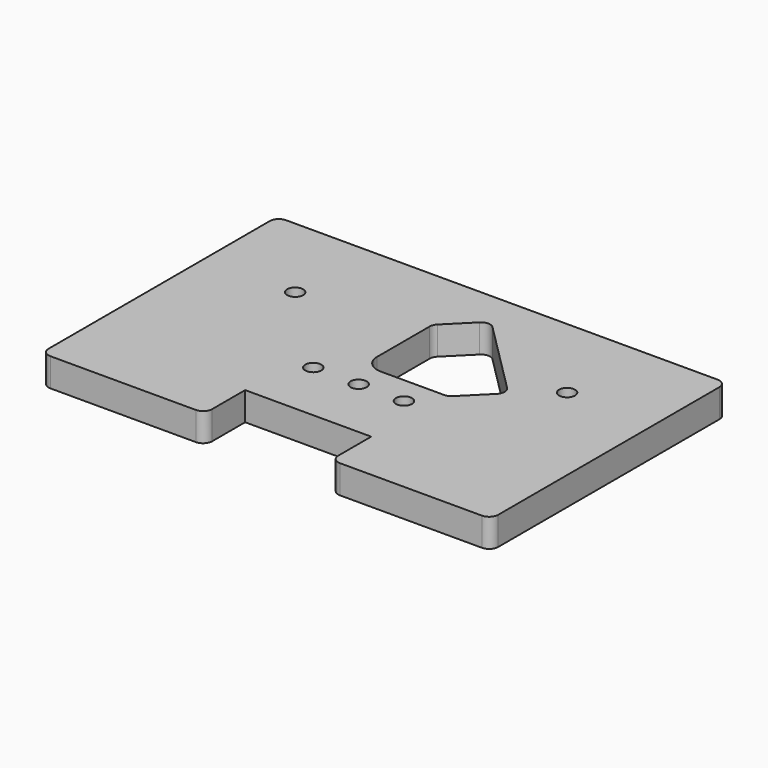
from build123d import *

# Parameters (mm, degrees)
F2_R     = 0.4490128061
F3_DEPTH = 1.5875
F4_R     = 0.508


# Not quite as in the source:
# - a length typed as a fraction of an inch, garbled in the dataset ("3 / 203.2 mm" for 3/8 in), is restored


with BuildPart() as f3:
    # F2 (on Top) → F3 (new body)
    with BuildSketch(Plane.XY):
        Polygon((9.1678125, 1.27), (9.1678125, 4.0878125), (16.2321875, 4.0878125), (16.2321875, 1.27), (25.2002304245, 1.27), (25.2002304245, 17.78), (0, 17.78), (0, 1.27), align=None)
        with Locations((10.16, 7.62)):
            Circle(F2_R, mode=Mode.SUBTRACT)
        with Locations((12.7, 7.62)):
            Circle(F2_R, mode=Mode.SUBTRACT)
        with Locations((15.24, 7.62)):
            Circle(F2_R, mode=Mode.SUBTRACT)
        with Locations((5.08, 12.7)):
            Circle(F2_R, mode=Mode.SUBTRACT)
        with BuildLine():
            Line((16.4718229778, 9.1678125), (12.7, 9.1678125))
            ThreePointArc((12.7, 9.1678125), (11.9984174905, 9.4584174905), (11.7078125, 10.16))
            Line((11.7078125, 10.16), (11.7078125, 14.0486225217))
            Line((11.7078125, 14.0486225217), (13.5308885435, 15.8716985652))
            Line((13.5308885435, 15.8716985652), (18.3532987932, 11.0492883154))
            Line((18.3532987932, 11.0492883154), (16.4718229778, 9.1678125))
        make_face(mode=Mode.SUBTRACT)
        with Locations((20.32, 12.7)):
            Circle(F2_R, mode=Mode.SUBTRACT)
    extrude(amount=F3_DEPTH)

    # F4
    f4_edges = [f3.edges().sort_by_distance(p)[0] for p in [
        (25.20023, 1.27, 0.79375),
        (16.232188, 1.27, 0.79375),
        (9.167813, 1.27, 0.79375),
        (0, 1.27, 0.79375),
        (0, 17.78, 0.79375),
        (25.20023, 17.78, 0.79375),
        (11.707813, 14.048623, 0.79375),
        (13.530889, 15.871699, 0.79375),
        (18.353299, 11.049288, 0.79375),
        (16.471823, 9.167813, 0.79375),
    ]]
    fillet(f4_edges, radius=F4_R)


solid = f3.part
